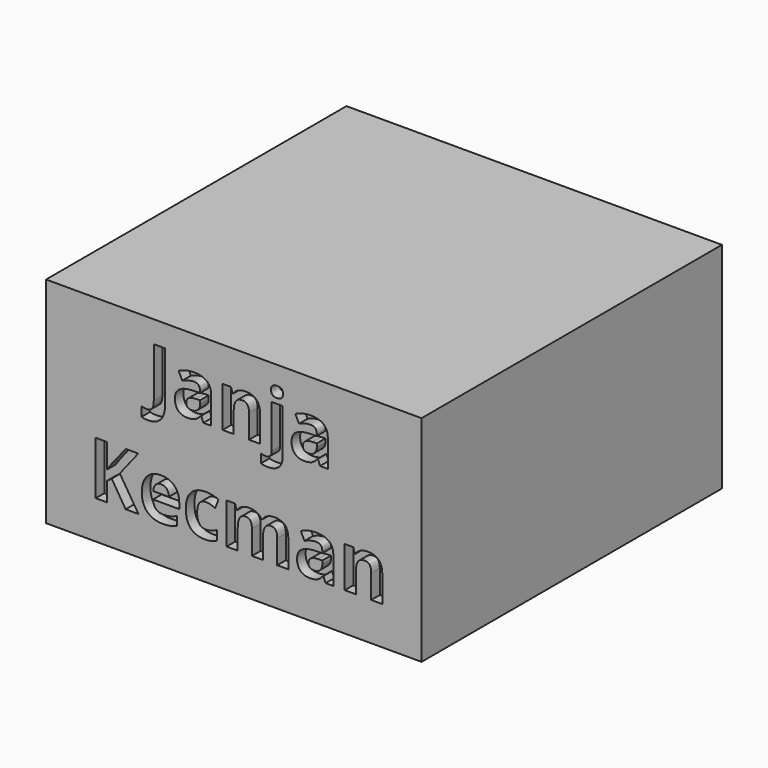
from build123d import *

# Parameters (mm, degrees)
F0_W         = 35
F0_H         = 35
F1_DEPTH     = 20
F2_TEXT_SIZE = 6.9444444444
F3_DEPTH     = 1


# Not quite as in the source:
# - Text() gives the source's letters only with a copy of the font that has no kerning and outlines rounded to 1/6400 em; it was checked with that copy


with BuildPart() as f1:
    # F0 (on Top) → F1 (new body)
    with BuildSketch(Plane.XY):
        with Locations((17.5, 17.5)):
            Rectangle(F0_W, F0_H)
    extrude(amount=F1_DEPTH)

    # F2 (on face) → F3 (cut)
    with BuildSketch(Plane.XZ):
        with Locations((9.4134114583, 13)):
            Text('Janja', F2_TEXT_SIZE, font='Open Sans', font_style=FontStyle.BOLD, text_align=(TextAlign.LEFT, TextAlign.BOTTOM))
        with Locations((4, 3.5555555556)):
            Text('Kecman', F2_TEXT_SIZE, font='Open Sans', font_style=FontStyle.BOLD, text_align=(TextAlign.LEFT, TextAlign.BOTTOM))
    extrude(amount=-F3_DEPTH, mode=Mode.SUBTRACT)


solid = f1.part
